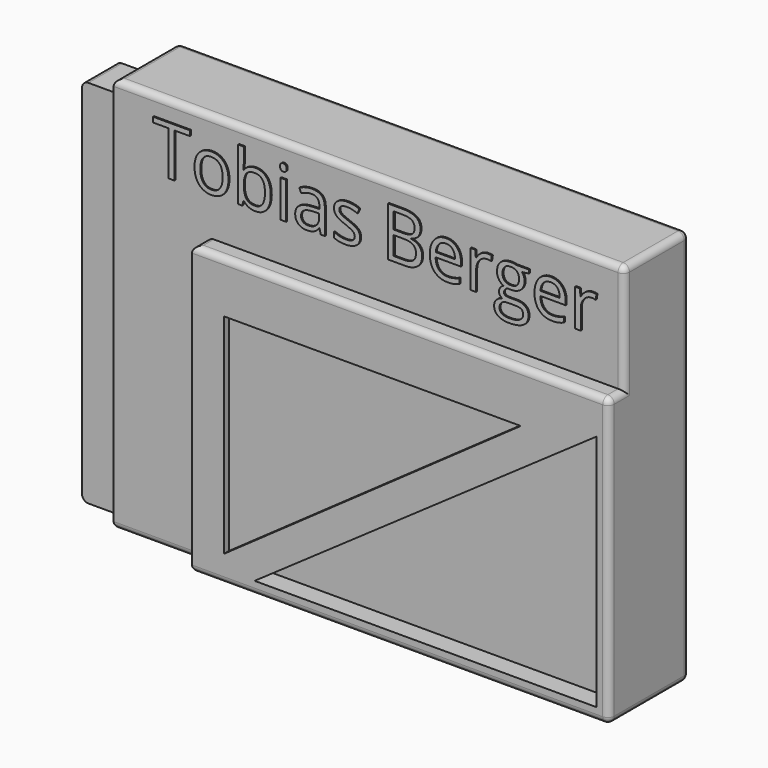
from build123d import *

# Parameters (mm, degrees)
F0_W           = 15
F0_H           = 15
F1_DEPTH       = 3.3
F2_W           = 78
F2_H           = 2
F3_DEPTH       = 3.3
F3_DEPTH_BACK  = 9.4
F4_DEPTH       = 2.5
F5_DEPTH       = 2.5
F7_W           = 2
F7_H           = 2
F7_W_2         = 5
F8_DEPTH       = 3
F9_DEPTH       = 2
F10_W          = 76
F10_H          = 58
F10_W_2        = 2
F11_DEPTH      = 2
F12_DEPTH      = 8
F12_DEPTH_BACK = 2
F13_TEXT_SIZE  = 10.8050078981
F14_DEPTH      = 0.2
F15_T1_DEPTH   = 66.8292834759
F15_T3_DEPTH   = 43
F15_T5_DEPTH   = 16
F15_T7_DEPTH   = 81.5
F15_T9_DEPTH   = 78
F15_T11_DEPTH  = 13.7
F15_T13_DEPTH  = 60
F15_T15_DEPTH  = 10.7
F15_T17_DEPTH  = 2
F15_T19_DEPTH  = 11.6
F15_T21_DEPTH  = 5.8
F15_T23_DEPTH  = 17.1707165241
F15_T25_DEPTH  = 1.8
F15_T27_DEPTH  = 5.5
F15_T29_DEPTH  = 14.2
F15_S33_W      = 1.02
F15_S33_H      = 1.02
F15_T34_DEPTH  = 1.02
F15_S39_W      = 1.02
F15_S39_H      = 1.02
F15_T40_DEPTH  = 1.02
F15_S45_W      = 1.02
F15_S45_H      = 1.02
F15_T46_DEPTH  = 1.02
F15_S51_W      = 1.02
F15_S51_H      = 1.02
F15_T52_DEPTH  = 1.02
F15_S57_W      = 1.02
F15_S57_H      = 1.02
F15_T58_DEPTH  = 1.02
F15_S63_W      = 1.02
F15_S63_H      = 1.02
F15_T64_DEPTH  = 1.02
F15_S69_W      = 1.02
F15_S69_H      = 1.02
F15_T70_DEPTH  = 1.02
F15_T77_DEPTH  = 18.5
F15_T81_DEPTH  = 4.5
F15_T88_DEPTH  = 5.5
F15_T92_DEPTH  = 17.1707165241


# Not quite as in the source:
# - a fillet or chamfer that OpenCascade refuses, or shapes differently, is made with other operations: its cross-section is extruded or revolved along the edge and cut away or added
# - a feature names something its author has since deleted; it is built from what else it names
# - Text() gives the source's letters only with a copy of the font that has no kerning and outlines rounded to 1/6400 em; it was checked with that copy


with BuildPart() as f1:
    # F0 (on Front) → F1 (new body, symmetric)
    with BuildSketch(Plane.XZ):
        Polygon((-87.6, -4.1635790914), (0, -4.1635790914), (0, 53.8364209086), (-87.6, 53.8364209086), (-87.6, 51.8364209086), (-2, 51.8364209086), (-2, -2.1635790914), (-87.6, -2.1635790914), align=None)
        with BuildLine():
            Line((-87.6, 12.8364209086), (-87.6, -2.1635790914))
            Line((-87.6, -2.1635790914), (-2, -2.1635790914))
            Line((-2, -2.1635790914), (-2, 51.8364209086))
            Line((-2, 51.8364209086), (-87.6, 51.8364209086))
            Line((-87.6, 51.8364209086), (-87.6, 27.8364209086))
            Line((-87.6, 27.8364209086), (-72.6, 27.8364209086))
            ThreePointArc((-72.6, 27.8364209086), (-65.1, 20.3364209086), (-72.6, 12.8364209086))
            Line((-72.6, 12.8364209086), (-87.6, 12.8364209086))
        make_face()
        with BuildLine():
            Line((-72.6, 27.8364209086), (-72.6, 12.8364209086))
            ThreePointArc((-72.6, 12.8364209086), (-65.1, 20.3364209086), (-72.6, 27.8364209086))
        make_face()
        with Locations((-80.1, 20.3364209086)):
            Rectangle(F0_W, F0_H)
    extrude(amount=F1_DEPTH, both=True)

    # F2 (on face) → F3 (join, two sides)
    with BuildSketch(Plane.XZ.offset(3.3)) as f3_sk:
        Polygon((-80, -4.1635790914), (0, -4.1635790914), (0, 53.8364209086), (-2, 53.8364209086), (-2, -2.1635790914), (-80, -2.1635790914), align=None)
        Polygon((-80, 51.8364209086), (-80, -2.1635790914), (-2, -2.1635790914), (-2, 53.8364209086), (-80, 53.8364209086), align=None)
        Polygon((-2, 53.8364209086), (0, 53.8364209086), (0, 57.8364209086), (-80, 57.8364209086), (-80, 55.8364209086), (-2, 55.8364209086), align=None)
        with Locations((-41, 54.8364209086)):
            Rectangle(F2_W, F2_H)
    extrude(amount=F3_DEPTH)
    extrude(f3_sk.sketch, amount=-F3_DEPTH_BACK)

    # F0 (on Front) → F4 (cut, symmetric)
    with BuildSketch(Plane.XZ):
        with BuildLine():
            Line((-87.6, 12.8364209086), (-87.6, -2.1635790914))
            Line((-87.6, -2.1635790914), (-2, -2.1635790914))
            Line((-2, -2.1635790914), (-2, 51.8364209086))
            Line((-2, 51.8364209086), (-87.6, 51.8364209086))
            Line((-87.6, 51.8364209086), (-87.6, 27.8364209086))
            Line((-87.6, 27.8364209086), (-72.6, 27.8364209086))
            ThreePointArc((-72.6, 27.8364209086), (-65.1, 20.3364209086), (-72.6, 12.8364209086))
            Line((-72.6, 12.8364209086), (-87.6, 12.8364209086))
        make_face()
        with BuildLine():
            Line((-72.6, 27.8364209086), (-72.6, 12.8364209086))
            ThreePointArc((-72.6, 12.8364209086), (-65.1, 20.3364209086), (-72.6, 27.8364209086))
        make_face()
        with Locations((-80.1, 20.3364209086)):
            Rectangle(F0_W, F0_H)
    extrude(amount=F4_DEPTH, both=True, mode=Mode.SUBTRACT)

    # F2 (on face) → F5 (cut)
    with BuildSketch(Plane.XZ.offset(3.3)):
        Polygon((-80, 51.8364209086), (-80, -2.1635790914), (-2, -2.1635790914), (-2, 53.8364209086), (-80, 53.8364209086), align=None)
        with Locations((-41, 54.8364209086)):
            Rectangle(F2_W, F2_H)
    extrude(amount=F5_DEPTH, mode=Mode.SUBTRACT)

    # F7 (on face) → F8 (join)
    with BuildSketch(Plane.XZ.offset(6.6)):
        with Locations((-1, -3.1635790914)):
            Rectangle(F7_W, F7_H)
        Polygon((-60.3292834759, -4.1635790914), (-2, -4.1635790914), (-2, -2.1635790914), (-55.527754128, -2.1635790914), (-60.3292834759, -2.1635790914), align=None)
        Polygon((-2, -2.1635790914), (0, -2.1635790914), (0, 38.8364209086), (-2, 38.8364209086), (-2, 35.1309031248), align=None)
        with Locations((-1, 39.8364209086)):
            Rectangle(F7_W, F7_H)
        Polygon((-5.192882847, 38.8364209086), (-2, 38.8364209086), (-2, 40.8364209086), (-60.3292834759, 40.8364209086), (-60.3292834759, 38.8364209086), align=None)
        with Locations((-62.8292834759, -3.1635790914)):
            Rectangle(F7_W_2, F7_H)
        Polygon((-65.3292834759, -2.1635790914), (-60.3292834759, -2.1635790914), (-60.3292834759, 0), (-60.3292834759, 32.7487625182), (-60.3292834759, 38.8364209086), (-65.3292834759, 38.8364209086), align=None)
        with Locations((-62.8292834759, 39.8364209086)):
            Rectangle(F7_W_2, F7_H)
        Polygon((-60.3292834759, 0), (-60.3292834759, -2.1635790914), (-55.527754128, -2.1635790914), (-2, 35.1309031248), (-2, 38.8364209086), (-5.192882847, 38.8364209086), (-13.8355837976, 32.7487625182), align=None)
        Polygon((-13.8355837976, 32.7487625182), (-5.192882847, 38.8364209086), (-60.3292834759, 38.8364209086), (-60.3292834759, 32.7487625182), align=None)
    extrude(amount=F8_DEPTH)

    # F7 (on face) → F9 (cut)
    with BuildSketch(Plane.XZ.offset(6.6)):
        Polygon((-65.3292834759, -2.1635790914), (-60.3292834759, -2.1635790914), (-60.3292834759, 0), (-60.3292834759, 32.7487625182), (-60.3292834759, 38.8364209086), (-65.3292834759, 38.8364209086), align=None)
        Polygon((-60.3292834759, 0), (-60.3292834759, -2.1635790914), (-55.527754128, -2.1635790914), (-2, 35.1309031248), (-2, 38.8364209086), (-5.192882847, 38.8364209086), (-13.8355837976, 32.7487625182), align=None)
        Polygon((-13.8355837976, 32.7487625182), (-5.192882847, 38.8364209086), (-60.3292834759, 38.8364209086), (-60.3292834759, 32.7487625182), align=None)
    extrude(amount=F9_DEPTH, mode=Mode.SUBTRACT)

    # F10 (on offset) → F11 (cut)
    with BuildSketch(Plane(origin=(0, 3.3, 0), x_dir=(-1, 0, 0), z_dir=(0, 1, 0))):
        with Locations((40, 26.836)):
            Rectangle(F10_W, F10_H)
        with Locations((79, 26.836)):
            Rectangle(F10_W_2, F10_H)
    extrude(amount=F11_DEPTH, mode=Mode.SUBTRACT)

    # F2 (on face) → F12 (cut, two sides)
    with BuildSketch(Plane.XZ.offset(3.3)) as f12_sk:
        with Locations((-41, 54.8364209086)):
            Rectangle(F2_W, F2_H)
    extrude(amount=-F12_DEPTH, mode=Mode.SUBTRACT)
    extrude(f12_sk.sketch, amount=F12_DEPTH_BACK, mode=Mode.SUBTRACT)

    # F13 (on face) → F14 (join)
    with BuildSketch(Plane.XZ.offset(6.6)):
        with Locations((-73.763474822, 47.0747947693)):
            Text('Tobias Berger', F13_TEXT_SIZE, font='Open Sans', text_align=(TextAlign.LEFT, TextAlign.BOTTOM))
    extrude(amount=F14_DEPTH)

    # F15: fillet of radius 1 on 20 edges, made by hand

    # F15_s2 → F15_t1 (cut)
    with BuildSketch(Plane.YZ.offset(-67.8292834759)):
        with BuildLine():
            ThreePointArc((-9.6, 39.8364209086), (-9.3071067812, 40.5435276898), (-8.6, 40.8364209086))
            Line((-8.6, 40.8364209086), (-9.6, 40.8364209086))
            Line((-9.6, 40.8364209086), (-9.6, 39.8364209086))
        make_face()
        with BuildLine():
            ThreePointArc((-8.6, -4.1635790914), (-9.3071067812, -3.8706858726), (-9.6, -3.1635790914))
            Line((-9.6, -3.1635790914), (-9.6, -4.1635790914))
            Line((-9.6, -4.1635790914), (-8.6, -4.1635790914))
        make_face()
    extrude(amount=F15_T1_DEPTH, mode=Mode.SUBTRACT)

    # F15_s4 → F15_t3 (cut)
    with BuildSketch(Plane.XY.offset(-3.1635790914)):
        with BuildLine():
            ThreePointArc((0, -8.6), (-0.2928932188, -9.3071067812), (-1, -9.6))
            Line((-1, -9.6), (0, -9.6))
            Line((0, -9.6), (0, -8.6))
        make_face()
    extrude(amount=F15_T3_DEPTH, mode=Mode.SUBTRACT)

    # F15_s6 → F15_t5 (cut)
    with BuildSketch(Plane.XY.offset(40.8364209086)):
        with BuildLine():
            ThreePointArc((0, -5.6), (-0.2928932188, -6.3071067812), (-1, -6.6))
            Line((-1, -6.6), (0, -6.6))
            Line((0, -6.6), (0, -5.6))
        make_face()
    extrude(amount=F15_T5_DEPTH, mode=Mode.SUBTRACT)

    # F15_s8 → F15_t7 (cut)
    with BuildSketch(Plane.YZ.offset(-82.5)):
        with BuildLine():
            ThreePointArc((-6.6, 56.8364209086), (-6.3071067812, 57.5435276898), (-5.6, 57.8364209086))
            Line((-5.6, 57.8364209086), (-6.6, 57.8364209086))
            Line((-6.6, 57.8364209086), (-6.6, 56.8364209086))
        make_face()
    extrude(amount=F15_T7_DEPTH, mode=Mode.SUBTRACT)

    # F15_s10 → F15_t9 (cut)
    with BuildSketch(Plane.YZ.offset(-79)):
        with BuildLine():
            ThreePointArc((6.1, 56.8364209086), (5.8071067812, 57.5435276898), (5.1, 57.8364209086))
            Line((5.1, 57.8364209086), (6.1, 57.8364209086))
            Line((6.1, 57.8364209086), (6.1, 56.8364209086))
        make_face()
        with BuildLine():
            ThreePointArc((5.1, -4.1635790914), (5.8071067812, -3.8706858726), (6.1, -3.1635790914))
            Line((6.1, -3.1635790914), (6.1, -4.1635790914))
            Line((6.1, -4.1635790914), (5.1, -4.1635790914))
        make_face()
    extrude(amount=F15_T9_DEPTH, mode=Mode.SUBTRACT)

    # F15_s12 → F15_t11 (cut)
    with BuildSketch(Plane.XZ.offset(-5.1)):
        with BuildLine():
            ThreePointArc((-1, -4.1635790914), (-0.2928932188, -3.8706858726), (0, -3.1635790914))
            Line((0, -3.1635790914), (0, -4.1635790914))
            Line((0, -4.1635790914), (-1, -4.1635790914))
        make_face()
    extrude(amount=F15_T11_DEPTH, mode=Mode.SUBTRACT)

    # F15_s14 → F15_t13 (cut)
    with BuildSketch(Plane.XY.offset(-3.1635790914)):
        with BuildLine():
            ThreePointArc((-1, 6.1), (-0.2928932188, 5.8071067812), (0, 5.1))
            Line((0, 5.1), (0, 6.1))
            Line((0, 6.1), (-1, 6.1))
        make_face()
        with BuildLine():
            ThreePointArc((-80, 5.1), (-79.7071067812, 5.8071067812), (-79, 6.1))
            Line((-79, 6.1), (-80, 6.1))
            Line((-80, 6.1), (-80, 5.1))
        make_face()
    extrude(amount=F15_T13_DEPTH, mode=Mode.SUBTRACT)

    # F15_s16 → F15_t15 (cut)
    with BuildSketch(Plane.XZ.offset(-5.1)):
        with BuildLine():
            ThreePointArc((0, 56.8364209086), (-0.2928932188, 57.5435276898), (-1, 57.8364209086))
            Line((-1, 57.8364209086), (0, 57.8364209086))
            Line((0, 57.8364209086), (0, 56.8364209086))
        make_face()
    extrude(amount=F15_T15_DEPTH, mode=Mode.SUBTRACT)

    # F15_s18 → F15_t17 (cut)
    with BuildSketch(Plane.XZ.offset(6.6)):
        with BuildLine():
            ThreePointArc((0, 39.8364209086), (-0.2928932188, 40.5435276898), (-1, 40.8364209086))
            Line((-1, 40.8364209086), (0, 40.8364209086))
            Line((0, 40.8364209086), (0, 39.8364209086))
        make_face()
    extrude(amount=F15_T17_DEPTH, mode=Mode.SUBTRACT)

    # F15_s20 → F15_t19 (cut)
    with BuildSketch(Plane.XZ.offset(-5.8)):
        with BuildLine():
            ThreePointArc((-86.6, -4.1635790914), (-87.3071067812, -3.8706858726), (-87.6, -3.1635790914))
            Line((-87.6, -3.1635790914), (-87.6, -4.1635790914))
            Line((-87.6, -4.1635790914), (-86.6, -4.1635790914))
        make_face()
        with BuildLine():
            ThreePointArc((-87.6, 52.8364209086), (-87.3071067812, 53.5435276898), (-86.6, 53.8364209086))
            Line((-86.6, 53.8364209086), (-87.6, 53.8364209086))
            Line((-87.6, 53.8364209086), (-87.6, 52.8364209086))
        make_face()
    extrude(amount=F15_T19_DEPTH, mode=Mode.SUBTRACT)

    # F15_s22 → F15_t21 (cut)
    with BuildSketch(Plane.XZ.offset(3.3)):
        with BuildLine():
            ThreePointArc((-79, -4.1635790914), (-79.7071067812, -3.8706858726), (-80, -3.1635790914))
            Line((-80, -3.1635790914), (-80, -4.1635790914))
            Line((-80, -4.1635790914), (-79, -4.1635790914))
        make_face()
    extrude(amount=F15_T21_DEPTH, mode=Mode.SUBTRACT)

    # F15_s24 → F15_t23 (cut)
    with BuildSketch(Plane.YZ.offset(-82.5)):
        with BuildLine():
            ThreePointArc((-5.6, -4.1635790914), (-6.3071067812, -3.8706858726), (-6.6, -3.1635790914))
            Line((-6.6, -3.1635790914), (-6.6, -4.1635790914))
            Line((-6.6, -4.1635790914), (-5.6, -4.1635790914))
        make_face()
    extrude(amount=F15_T23_DEPTH, mode=Mode.SUBTRACT)

    # F15_s26 → F15_t25 (cut)
    with BuildSketch(Plane.XZ.offset(-5.1)):
        with BuildLine():
            ThreePointArc((-79, -4.1635790914), (-79.7071067812, -3.8706858726), (-80, -3.1635790914))
            Line((-80, -3.1635790914), (-80, -4.1635790914))
            Line((-80, -4.1635790914), (-79, -4.1635790914))
        make_face()
    extrude(amount=F15_T25_DEPTH, mode=Mode.SUBTRACT)

    # F15_s28 → F15_t27 (cut)
    with BuildSketch(Plane.XZ.offset(6.6)):
        with BuildLine():
            ThreePointArc((-64.3292834759, -4.1635790914), (-65.0363902571, -3.8706858726), (-65.3292834759, -3.1635790914))
            Line((-65.3292834759, -3.1635790914), (-65.3292834759, -4.1635790914))
            Line((-65.3292834759, -4.1635790914), (-64.3292834759, -4.1635790914))
        make_face()
        with BuildLine():
            ThreePointArc((-65.3292834759, 39.8364209086), (-65.0363902571, 40.5435276898), (-64.3292834759, 40.8364209086))
            Line((-64.3292834759, 40.8364209086), (-65.3292834759, 40.8364209086))
            Line((-65.3292834759, 40.8364209086), (-65.3292834759, 39.8364209086))
        make_face()
    extrude(amount=F15_T27_DEPTH, mode=Mode.SUBTRACT)

    # F15_s30 → F15_t29 (cut)
    with BuildSketch(Plane.XZ.offset(-5.1)):
        with BuildLine():
            ThreePointArc((-80, 56.8364209086), (-79.7071067812, 57.5435276898), (-79, 57.8364209086))
            Line((-79, 57.8364209086), (-80, 57.8364209086))
            Line((-80, 57.8364209086), (-80, 56.8364209086))
        make_face()
    extrude(amount=F15_T29_DEPTH, mode=Mode.SUBTRACT)


with BuildPart() as f15_tool32:
    # F15_s33 → F15_t34 (new body)
    with BuildSketch(Plane.XY.offset(39.8364209086)):
        with Locations((-0.49, -9.11)):
            Rectangle(F15_S33_W, F15_S33_H)
    extrude(amount=F15_T34_DEPTH)

    # F15_s35 → F15_t36 (revolve, cut)
    with BuildSketch(Plane(origin=(-1, -8.6, 39.8364209086), x_dir=(-0.7071067812, 0.7071067812, 0), z_dir=(0.7071067812, 0.7071067812, 0))):
        with BuildLine():
            ThreePointArc((0, -1), (1, 0), (0, 1))
            Line((0, 1), (0, -1))
        make_face()
    revolve(axis=Axis((-1, -8.6, 39.8364209086), (0, 0, 1)), mode=Mode.SUBTRACT)


with BuildPart() as f1_1:
    add(f1.part)

    # F15_t31: cut F15_tool32
    add(f15_tool32.part, mode=Mode.SUBTRACT)


with BuildPart() as f15_tool38:
    # F15_s39 → F15_t40 (new body)
    with BuildSketch(Plane.XY.offset(-3.1635790914)):
        with Locations((-0.49, -9.11)):
            Rectangle(F15_S39_W, F15_S39_H)
    extrude(amount=-F15_T40_DEPTH)

    # F15_s41 → F15_t42 (revolve, cut)
    with BuildSketch(Plane(origin=(-1, -8.6, -3.1635790914), x_dir=(-0.7071067812, 0.7071067812, 0), z_dir=(-0.7071067812, -0.7071067812, 0))):
        with BuildLine():
            ThreePointArc((0, -1), (1, 0), (0, 1))
            Line((0, 1), (0, -1))
        make_face()
    revolve(axis=Axis((-1, -8.6, -3.1635790914), (0, 0, -1)), mode=Mode.SUBTRACT)


with BuildPart() as f1_2:
    add(f1_1.part)

    # F15_t37: cut F15_tool38
    add(f15_tool38.part, mode=Mode.SUBTRACT)


with BuildPart() as f15_tool44:
    # F15_s45 → F15_t46 (new body)
    with BuildSketch(Plane.XZ.offset(5.6)):
        with Locations((-0.49, 57.3464209086)):
            Rectangle(F15_S45_W, F15_S45_H)
    extrude(amount=F15_T46_DEPTH)

    # F15_s47 → F15_t48 (revolve, cut)
    with BuildSketch(Plane(origin=(-1, -5.6, 56.8364209086), x_dir=(-0.7071067812, 0, -0.7071067812), z_dir=(-0.7071067812, 0, 0.7071067812))):
        with BuildLine():
            ThreePointArc((0, -1), (1, 0), (0, 1))
            Line((0, 1), (0, -1))
        make_face()
    revolve(axis=Axis((-1, -5.6, 56.8364209086), (0, -1, 0)), mode=Mode.SUBTRACT)


with BuildPart() as f1_3:
    add(f1_2.part)

    # F15_t43: cut F15_tool44
    add(f15_tool44.part, mode=Mode.SUBTRACT)


with BuildPart() as f15_tool50:
    # F15_s51 → F15_t52 (new body)
    with BuildSketch(Plane.XY.offset(56.8364209086)):
        with Locations((-0.49, 5.61)):
            Rectangle(F15_S51_W, F15_S51_H)
    extrude(amount=F15_T52_DEPTH)

    # F15_s53 → F15_t54 (revolve, cut)
    with BuildSketch(Plane(origin=(-1, 5.1, 56.8364209086), x_dir=(-0.7071067812, -0.7071067812, 0), z_dir=(-0.7071067812, 0.7071067812, 0))):
        with BuildLine():
            ThreePointArc((0, -1), (1, 0), (0, 1))
            Line((0, 1), (0, -1))
        make_face()
    revolve(axis=Axis((-1, 5.1, 56.8364209086), (0, 0, 1)), mode=Mode.SUBTRACT)


with BuildPart() as f1_4:
    add(f1_3.part)

    # F15_t49: cut F15_tool50
    add(f15_tool50.part, mode=Mode.SUBTRACT)


with BuildPart() as f15_tool56:
    # F15_s57 → F15_t58 (new body)
    with BuildSketch(Plane.XY.offset(56.8364209086)):
        with Locations((-79.51, 5.61)):
            Rectangle(F15_S57_W, F15_S57_H)
    extrude(amount=F15_T58_DEPTH)

    # F15_s59 → F15_t60 (revolve, cut)
    with BuildSketch(Plane(origin=(-79, 5.1, 56.8364209086), x_dir=(0.7071067812, -0.7071067812, 0), z_dir=(-0.7071067812, -0.7071067812, 0))):
        with BuildLine():
            ThreePointArc((0, -1), (1, 0), (0, 1))
            Line((0, 1), (0, -1))
        make_face()
    revolve(axis=Axis((-79, 5.1, 56.8364209086), (0, 0, 1)), mode=Mode.SUBTRACT)


with BuildPart() as f1_5:
    add(f1_4.part)

    # F15_t55: cut F15_tool56
    add(f15_tool56.part, mode=Mode.SUBTRACT)


with BuildPart() as f15_tool62:
    # F15_s63 → F15_t64 (new body)
    with BuildSketch(Plane.XY.offset(-3.1635790914)):
        with Locations((-79.51, 5.61)):
            Rectangle(F15_S63_W, F15_S63_H)
    extrude(amount=-F15_T64_DEPTH)

    # F15_s65 → F15_t66 (revolve, cut)
    with BuildSketch(Plane(origin=(-79, 5.1, -3.1635790914), x_dir=(0.7071067812, -0.7071067812, 0), z_dir=(0.7071067812, 0.7071067812, 0))):
        with BuildLine():
            ThreePointArc((0, -1), (1, 0), (0, 1))
            Line((0, 1), (0, -1))
        make_face()
    revolve(axis=Axis((-79, 5.1, -3.1635790914), (0, 0, -1)), mode=Mode.SUBTRACT)


with BuildPart() as f1_6:
    add(f1_5.part)

    # F15_t61: cut F15_tool62
    add(f15_tool62.part, mode=Mode.SUBTRACT)


with BuildPart() as f15_tool68:
    # F15_s69 → F15_t70 (new body)
    with BuildSketch(Plane.XY.offset(-3.1635790914)):
        with Locations((-0.49, 5.61)):
            Rectangle(F15_S69_W, F15_S69_H)
    extrude(amount=-F15_T70_DEPTH)

    # F15_s71 → F15_t72 (revolve, cut)
    with BuildSketch(Plane(origin=(-1, 5.1, -3.1635790914), x_dir=(-0.7071067812, -0.7071067812, 0), z_dir=(0.7071067812, -0.7071067812, 0))):
        with BuildLine():
            ThreePointArc((0, -1), (1, 0), (0, 1))
            Line((0, 1), (0, -1))
        make_face()
    revolve(axis=Axis((-1, 5.1, -3.1635790914), (0, 0, -1)), mode=Mode.SUBTRACT)


with BuildPart() as f1_7:
    add(f1_6.part)

    # F15_t67: cut F15_tool68
    add(f15_tool68.part, mode=Mode.SUBTRACT)


with BuildPart() as f15_tool75:
    # F15_s76 → F15_t77 (new body)
    with BuildSketch(Plane.XY.offset(38.3364209086)):
        with BuildLine():
            ThreePointArc((0, -5.6), (-0.2928932188, -6.3071067812), (-1, -6.6))
            Line((-1, -6.6), (0, -6.6))
            Line((0, -6.6), (0, -5.6))
        make_face()
    extrude(amount=F15_T77_DEPTH)

    split(bisect_by=Plane.XY.offset(40.8364209086), keep=Keep.BOTTOM)


with BuildPart() as f15_tool79:
    # F15_s80 → F15_t81 (new body)
    with BuildSketch(Plane.XZ.offset(4.1)):
        with BuildLine():
            ThreePointArc((0, 39.8364209086), (-0.2928932188, 40.5435276898), (-1, 40.8364209086))
            Line((-1, 40.8364209086), (0, 40.8364209086))
            Line((0, 40.8364209086), (0, 39.8364209086))
        make_face()
    extrude(amount=F15_T81_DEPTH)

    split(bisect_by=Plane.XZ.offset(6.6), keep=Keep.BOTTOM)


with BuildPart() as f15_tool75_1:
    add(f15_tool75.part)

    # F15_t83: intersect F15_tool79
    add(f15_tool79.part, mode=Mode.INTERSECT)


with BuildPart() as f1_8:
    add(f1_7.part)

    # F15_t73: cut F15_tool75
    add(f15_tool75_1.part, mode=Mode.SUBTRACT)


with BuildPart() as f15_tool86:
    # F15_s87 → F15_t88 (new body)
    with BuildSketch(Plane.XZ.offset(4.1)):
        with BuildLine():
            ThreePointArc((-64.3292834759, -4.1635790914), (-65.0363902571, -3.8706858726), (-65.3292834759, -3.1635790914))
            Line((-65.3292834759, -3.1635790914), (-65.3292834759, -4.1635790914))
            Line((-65.3292834759, -4.1635790914), (-64.3292834759, -4.1635790914))
        make_face()
    extrude(amount=F15_T88_DEPTH)

    split(bisect_by=Plane.XZ.offset(6.6), keep=Keep.BOTTOM)


with BuildPart() as f15_tool90:
    # F15_s91 → F15_t92 (new body)
    with BuildSketch(Plane.YZ.offset(-80)):
        with BuildLine():
            ThreePointArc((-5.6, -4.1635790914), (-6.3071067812, -3.8706858726), (-6.6, -3.1635790914))
            Line((-6.6, -3.1635790914), (-6.6, -4.1635790914))
            Line((-6.6, -4.1635790914), (-5.6, -4.1635790914))
        make_face()
    extrude(amount=F15_T92_DEPTH)

    split(bisect_by=Plane.YZ.offset(-65.3292834759), keep=Keep.TOP)


with BuildPart() as f15_tool86_1:
    add(f15_tool86.part)

    # F15_t94: intersect F15_tool90
    add(f15_tool90.part, mode=Mode.INTERSECT)


with BuildPart() as f1_9:
    add(f1_8.part)

    # F15_t84: cut F15_tool86
    add(f15_tool86_1.part, mode=Mode.SUBTRACT)


solid = f1_9.part
